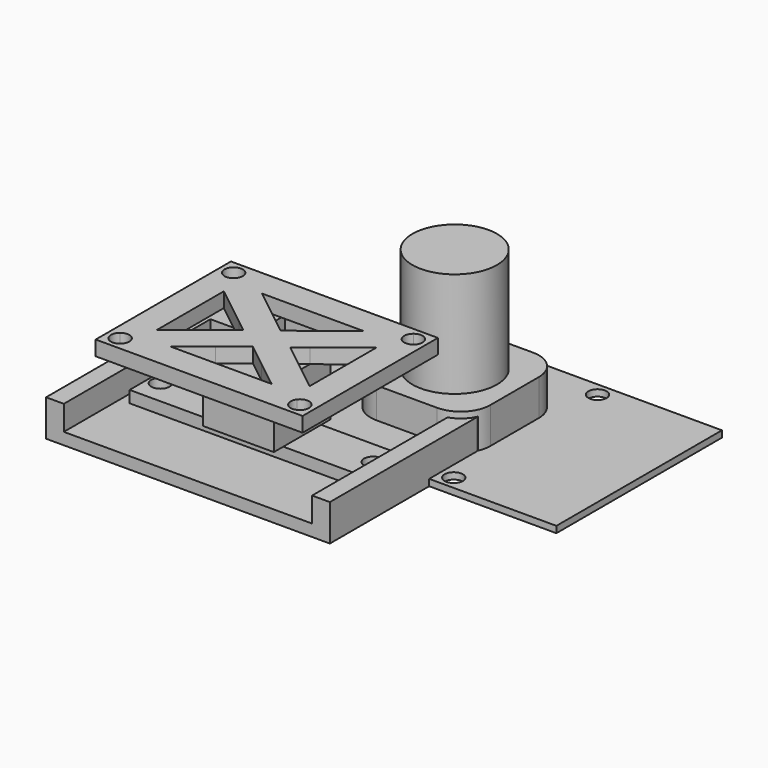
from build123d import *

# Parameters (mm, degrees)
F0_W      = 45.5
F0_H      = 35
F0_R      = 1.55
F1_DEPTH  = 1.1
F0_R_2    = 7.15
F2_DEPTH  = 7.2
F3_DEPTH  = 25
F4_R      = 1.55
F5_DEPTH  = 2
F6_DEPTH  = 6.175
F7_W      = 40
F7_H      = 8
F7_R      = 1.55
F8_DEPTH  = 4
F9_W      = 12
F9_H      = 2
F9_H_2    = 8
F10_DEPTH = 10
F11_W     = 35
F11_H     = 28.6
F12_DEPTH = 2.5


with BuildPart() as f1:
    # F0 (on Top) → F1 (new body)
    with BuildSketch(Plane.XY):
        with Locations((22.75, 17.5)):
            Rectangle(F0_W, F0_H)
        with Locations((2.3, 2.3)):
            Circle(F0_R, mode=Mode.SUBTRACT)
        with Locations((26.3, 2.3)):
            Circle(F0_R, mode=Mode.SUBTRACT)
        with BuildLine():
            Line((9.175, 27.625), (19.425, 27.625))
            ThreePointArc((19.425, 27.625), (22.9605339059, 26.1605339059), (24.425, 22.625))
            Line((24.425, 22.625), (24.425, 12.375))
            ThreePointArc((24.425, 12.375), (22.9605339059, 8.8394660941), (19.425, 7.375))
            Line((19.425, 7.375), (9.175, 7.375))
            ThreePointArc((9.175, 7.375), (5.6394660941, 8.8394660941), (4.175, 12.375))
            Line((4.175, 12.375), (4.175, 22.625))
            ThreePointArc((4.175, 22.625), (5.6394660941, 26.1605339059), (9.175, 27.625))
        make_face(mode=Mode.SUBTRACT)
        with Locations((2.3, 32.7)):
            Circle(F0_R, mode=Mode.SUBTRACT)
        with Locations((26.3, 32.7)):
            Circle(F0_R, mode=Mode.SUBTRACT)
    extrude(amount=F1_DEPTH)

    # F0 (on Top) → F2 (join)
    with BuildSketch(Plane.XY):
        with BuildLine():
            ThreePointArc((24.425, 22.625), (22.9605339059, 26.1605339059), (19.425, 27.625))
            Line((19.425, 27.625), (9.175, 27.625))
            ThreePointArc((9.175, 27.625), (5.6394660941, 26.1605339059), (4.175, 22.625))
            Line((4.175, 22.625), (4.175, 12.375))
            ThreePointArc((4.175, 12.375), (5.6394660941, 8.8394660941), (9.175, 7.375))
            Line((9.175, 7.375), (19.425, 7.375))
            ThreePointArc((19.425, 7.375), (22.9605339059, 8.8394660941), (24.425, 12.375))
            Line((24.425, 12.375), (24.425, 22.625))
        make_face()
        with Locations((14.3, 17.5)):
            Circle(F0_R_2, mode=Mode.SUBTRACT)
    extrude(amount=F2_DEPTH)

    # F0 (on Top) → F3 (join)
    with BuildSketch(Plane.XY):
        with Locations((14.3, 17.5)):
            Circle(F0_R_2)
    extrude(amount=F3_DEPTH)


with BuildPart() as f5:
    # F4 (on Top) → F5 (new body)
    with BuildSketch(Plane.XY):
        Polygon((-21.0177182555, 10), (-21.0177182555, -21), (20.9822817445, -21), (20.9822817445, 10), (13.9822817445, 10), (13.9822817445, 17), (-14.0177182555, 17), (-14.0177182555, 10), align=None)
        with Locations((-18.0177182555, 0)):
            Circle(F4_R, mode=Mode.SUBTRACT)
        with Locations((17.9822817445, 0)):
            Circle(F4_R, mode=Mode.SUBTRACT)
    extrude(amount=F5_DEPTH)

    # F4 (on Top) → F6 (join)
    with BuildSketch(Plane.XY):
        with BuildLine():
            Line((13.9822817445, 20), (-14.0177182555, 20))
            ThreePointArc((-14.0177182555, 20), (-21.0887860674, 17.0710678119), (-24.0177182555, 10))
            Line((-24.0177182555, 10), (-24.0177182555, -21))
            Line((-24.0177182555, -21), (-21.0177182555, -21))
            Line((-21.0177182555, -21), (-21.0177182555, 10))
            ThreePointArc((-21.0177182555, 10), (-18.9674657238, 14.9497474683), (-14.0177182555, 17))
            Line((-14.0177182555, 17), (13.9822817445, 17))
            ThreePointArc((13.9822817445, 17), (18.9320292128, 14.9497474683), (20.9822817445, 10))
            Line((20.9822817445, 10), (20.9822817445, -21))
            Line((20.9822817445, -21), (23.9822817445, -21))
            Line((23.9822817445, -21), (23.9822817445, 10))
            ThreePointArc((23.9822817445, 10), (21.0533495563, 17.0710678119), (13.9822817445, 20))
        make_face()
        with BuildLine():
            Line((13.9822817445, 10), (20.9822817445, 10))
            ThreePointArc((20.9822817445, 10), (18.9320292128, 14.9497474683), (13.9822817445, 17))
            Line((13.9822817445, 17), (13.9822817445, 10))
        make_face()
        with BuildLine():
            ThreePointArc((-14.0177182555, 17), (-18.9674657238, 14.9497474683), (-21.0177182555, 10))
            Line((-21.0177182555, 10), (-14.0177182555, 10))
            Line((-14.0177182555, 10), (-14.0177182555, 17))
        make_face()
    extrude(amount=F6_DEPTH)


with BuildPart() as f8:
    # F7 (on Top) → F8 (new body)
    with BuildSketch(Plane.XY):
        with Locations((0.6692926586, -5.1978348792)):
            Rectangle(F7_W, F7_H)
        with Locations((-17.3307073414, -5.1978348792)):
            Circle(F7_R, mode=Mode.SUBTRACT)
        with Locations((18.6692926586, -5.1978348792)):
            Circle(F7_R, mode=Mode.SUBTRACT)
    extrude(amount=F8_DEPTH)

    # F9 (on face) → F10 (join)
    with BuildSketch(Plane.XY.offset(4)):
        with Locations((0.6692926586, -0.1978348792)):
            Rectangle(F9_W, F9_H)
        with Locations((0.6692926586, -10.1978348792)):
            Rectangle(F9_W, F9_H)
        with Locations((0.6692926586, -5.1978348792)):
            Rectangle(F9_W, F9_H_2)
    extrude(amount=F10_DEPTH)

    # F11 (on face) → F12 (join)
    with BuildSketch(Plane.XY.offset(14)):
        with Locations((0.6692926586, -5.1978348792)):
            Rectangle(F11_W, F11_H)
        with BuildLine():
            Line((-12.2307073414, -12.2517855581), (-12.2307073414, 1.8561157997))
            Line((-12.2307073414, 1.8561157997), (-16.0531033423, 4.8737968531))
            Line((-16.0531033423, 4.8737968531), (-15.4911559887, 5.5855968343))
            ThreePointArc((-15.4911559887, 5.5855968343), (-15.747275628, 7.7626137681), (-13.5702586941, 8.0187334074))
            Line((-13.5702586941, 8.0187334074), (-13.1055254777, 8.6073954816))
            Line((-13.1055254777, 8.6073954816), (-7.9055670208, 4.5021651208))
            Line((-7.9055670208, 4.5021651208), (9.2441523379, 4.5021651208))
            Line((9.2441523379, 4.5021651208), (14.4441107948, 8.6073954816))
            Line((14.4441107948, 8.6073954816), (14.9088440113, 8.0187334074))
            ThreePointArc((14.9088440113, 8.0187334074), (16.5452381433, 8.1970119589), (17.4192926586, 6.8021651208))
            ThreePointArc((17.4192926586, 6.8021651208), (17.2641394966, 6.1262196361), (16.8297413059, 5.5855968343))
            Line((16.8297413059, 5.5855968343), (17.3916886594, 4.8737968531))
            Line((17.3916886594, 4.8737968531), (13.5692926586, 1.8561157997))
            Line((13.5692926586, 1.8561157997), (13.5692926586, -12.2517855581))
            Line((13.5692926586, -12.2517855581), (17.3916886594, -15.2694666114))
            Line((17.3916886594, -15.2694666114), (16.8297413059, -15.9812665926))
            ThreePointArc((16.8297413059, -15.9812665926), (17.2641394966, -16.5218893944), (17.4192926586, -17.1978348792))
            ThreePointArc((17.4192926586, -17.1978348792), (16.5452381433, -18.5926817172), (14.9088440113, -18.4144031657))
            Line((14.9088440113, -18.4144031657), (14.4441107948, -19.0030652399))
            Line((14.4441107948, -19.0030652399), (9.2441523379, -14.8978348792))
            Line((9.2441523379, -14.8978348792), (-7.9055670208, -14.8978348792))
            Line((-7.9055670208, -14.8978348792), (-13.1055254777, -19.0030652399))
            Line((-13.1055254777, -19.0030652399), (-13.5702586941, -18.4144031657))
            ThreePointArc((-13.5702586941, -18.4144031657), (-15.747275628, -18.1582835265), (-15.4911559887, -15.9812665926))
            Line((-15.4911559887, -15.9812665926), (-16.0531033423, -15.2694666114))
            Line((-16.0531033423, -15.2694666114), (-12.2307073414, -12.2517855581))
        make_face(mode=Mode.SUBTRACT)
        Polygon((12.9559593252, 4.5021651208), (9.2441523379, 4.5021651208), (4.5574856712, 0.8021651208), (6.6692926586, 0.8021651208), (6.6692926586, -0.4609927739), align=None)
        Polygon((13.5692926586, 4.5021651208), (12.9559593252, 4.5021651208), (6.6692926586, -0.4609927739), (6.6692926586, -3.5912526213), (13.5692926586, 1.8561157997), align=None)
        Polygon((-5.3307073414, 0.8021651208), (-5.3307073414, -0.4609927739), (0.6692926586, -5.1978348792), (6.6692926586, -0.4609927739), (6.6692926586, 0.8021651208), (4.5574856712, 0.8021651208), (0.6692926586, -2.2674609418), (-3.2189003541, 0.8021651208), align=None)
        Polygon((6.6692926586, -0.4609927739), (0.6692926586, -5.1978348792), (6.6692926586, -9.9346769844), (6.6692926586, -6.804417137), (4.6342884653, -5.1978348792), (6.6692926586, -3.5912526213), align=None)
        Polygon((-7.9055670208, 4.5021651208), (-11.6173740081, 4.5021651208), (-5.3307073414, -0.4609927739), (-5.3307073414, 0.8021651208), (-3.2189003541, 0.8021651208), align=None)
        Polygon((-11.6173740081, 4.5021651208), (-12.2307073414, 4.5021651208), (-12.2307073414, 1.8561157997), (-5.3307073414, -3.5912526213), (-5.3307073414, -0.4609927739), align=None)
        Polygon((-5.3307073414, -6.804417137), (-12.2307073414, -12.2517855581), (-12.2307073414, -14.8978348792), (-11.6173740081, -14.8978348792), (-5.3307073414, -9.9346769844), align=None)
        Polygon((-5.3307073414, -9.9346769844), (-11.6173740081, -14.8978348792), (-7.9055670208, -14.8978348792), (-3.2189003541, -11.1978348792), (-5.3307073414, -11.1978348792), align=None)
        Polygon((6.6692926586, -9.9346769844), (0.6692926586, -5.1978348792), (-5.3307073414, -9.9346769844), (-5.3307073414, -11.1978348792), (-3.2189003541, -11.1978348792), (0.6692926586, -8.1282088165), (4.5574856712, -11.1978348792), (6.6692926586, -11.1978348792), align=None)
        Polygon((-5.3307073414, -0.4609927739), (-5.3307073414, -3.5912526213), (-3.2957031482, -5.1978348792), (-5.3307073414, -6.804417137), (-5.3307073414, -9.9346769844), (0.6692926586, -5.1978348792), align=None)
        Polygon((12.9559593252, -14.8978348792), (6.6692926586, -9.9346769844), (6.6692926586, -11.1978348792), (4.5574856712, -11.1978348792), (9.2441523379, -14.8978348792), align=None)
        Polygon((6.6692926586, -6.804417137), (6.6692926586, -9.9346769844), (12.9559593252, -14.8978348792), (13.5692926586, -14.8978348792), (13.5692926586, -12.2517855581), align=None)
        with BuildLine():
            Line((-12.2307073414, 1.8561157997), (-12.2307073414, 4.5021651208))
            Line((-12.2307073414, 4.5021651208), (-11.6173740081, 4.5021651208))
            Line((-11.6173740081, 4.5021651208), (-13.3141390549, 5.8417164735))
            ThreePointArc((-13.3141390549, 5.8417164735), (-14.3496034077, 5.2627816841), (-15.4911559887, 5.5855968343))
            Line((-15.4911559887, 5.5855968343), (-16.0531033423, 4.8737968531))
            Line((-16.0531033423, 4.8737968531), (-12.2307073414, 1.8561157997))
        make_face()
        with BuildLine():
            Line((-13.3141390549, 5.8417164735), (-11.6173740081, 4.5021651208))
            Line((-11.6173740081, 4.5021651208), (-7.9055670208, 4.5021651208))
            Line((-7.9055670208, 4.5021651208), (-13.1055254777, 8.6073954816))
            Line((-13.1055254777, 8.6073954816), (-13.5702586941, 8.0187334074))
            ThreePointArc((-13.5702586941, 8.0187334074), (-13.1358605034, 7.4781106056), (-12.9807073414, 6.8021651208))
            ThreePointArc((-12.9807073414, 6.8021651208), (-13.0664360475, 6.2938250989), (-13.3141390549, 5.8417164735))
        make_face()
        with BuildLine():
            Line((-12.2307073414, -14.8978348792), (-12.2307073414, -12.2517855581))
            Line((-12.2307073414, -12.2517855581), (-16.0531033423, -15.2694666114))
            Line((-16.0531033423, -15.2694666114), (-15.4911559887, -15.9812665926))
            ThreePointArc((-15.4911559887, -15.9812665926), (-14.3496034077, -15.6584514425), (-13.3141390549, -16.2373862319))
            Line((-13.3141390549, -16.2373862319), (-11.6173740081, -14.8978348792))
            Line((-11.6173740081, -14.8978348792), (-12.2307073414, -14.8978348792))
        make_face()
        with BuildLine():
            Line((-7.9055670208, -14.8978348792), (-11.6173740081, -14.8978348792))
            Line((-11.6173740081, -14.8978348792), (-13.3141390549, -16.2373862319))
            ThreePointArc((-13.3141390549, -16.2373862319), (-13.0664360475, -16.6894948572), (-12.9807073414, -17.1978348792))
            ThreePointArc((-12.9807073414, -17.1978348792), (-13.1358605034, -17.8737803639), (-13.5702586941, -18.4144031657))
            Line((-13.5702586941, -18.4144031657), (-13.1055254777, -19.0030652399))
            Line((-13.1055254777, -19.0030652399), (-7.9055670208, -14.8978348792))
        make_face()
        with BuildLine():
            Line((14.652724372, -16.2373862319), (12.9559593252, -14.8978348792))
            Line((12.9559593252, -14.8978348792), (9.2441523379, -14.8978348792))
            Line((9.2441523379, -14.8978348792), (14.4441107948, -19.0030652399))
            Line((14.4441107948, -19.0030652399), (14.9088440113, -18.4144031657))
            ThreePointArc((14.9088440113, -18.4144031657), (14.3299092219, -17.3789388129), (14.652724372, -16.2373862319))
        make_face()
        with BuildLine():
            Line((13.5692926586, -14.8978348792), (12.9559593252, -14.8978348792))
            Line((12.9559593252, -14.8978348792), (14.652724372, -16.2373862319))
            ThreePointArc((14.652724372, -16.2373862319), (15.6881887248, -15.6584514425), (16.8297413059, -15.9812665926))
            Line((16.8297413059, -15.9812665926), (17.3916886594, -15.2694666114))
            Line((17.3916886594, -15.2694666114), (13.5692926586, -12.2517855581))
            Line((13.5692926586, -12.2517855581), (13.5692926586, -14.8978348792))
        make_face()
        with BuildLine():
            Line((14.4441107948, 8.6073954816), (9.2441523379, 4.5021651208))
            Line((9.2441523379, 4.5021651208), (12.9559593252, 4.5021651208))
            Line((12.9559593252, 4.5021651208), (14.652724372, 5.8417164735))
            ThreePointArc((14.652724372, 5.8417164735), (14.3299092219, 6.9832690546), (14.9088440113, 8.0187334074))
            Line((14.9088440113, 8.0187334074), (14.4441107948, 8.6073954816))
        make_face()
        with BuildLine():
            Line((14.652724372, 5.8417164735), (12.9559593252, 4.5021651208))
            Line((12.9559593252, 4.5021651208), (13.5692926586, 4.5021651208))
            Line((13.5692926586, 4.5021651208), (13.5692926586, 1.8561157997))
            Line((13.5692926586, 1.8561157997), (17.3916886594, 4.8737968531))
            Line((17.3916886594, 4.8737968531), (16.8297413059, 5.5855968343))
            ThreePointArc((16.8297413059, 5.5855968343), (15.6881887248, 5.2627816841), (14.652724372, 5.8417164735))
        make_face()
    extrude(amount=F12_DEPTH)


solid = Compound([f1.part, f5.part, f8.part])
